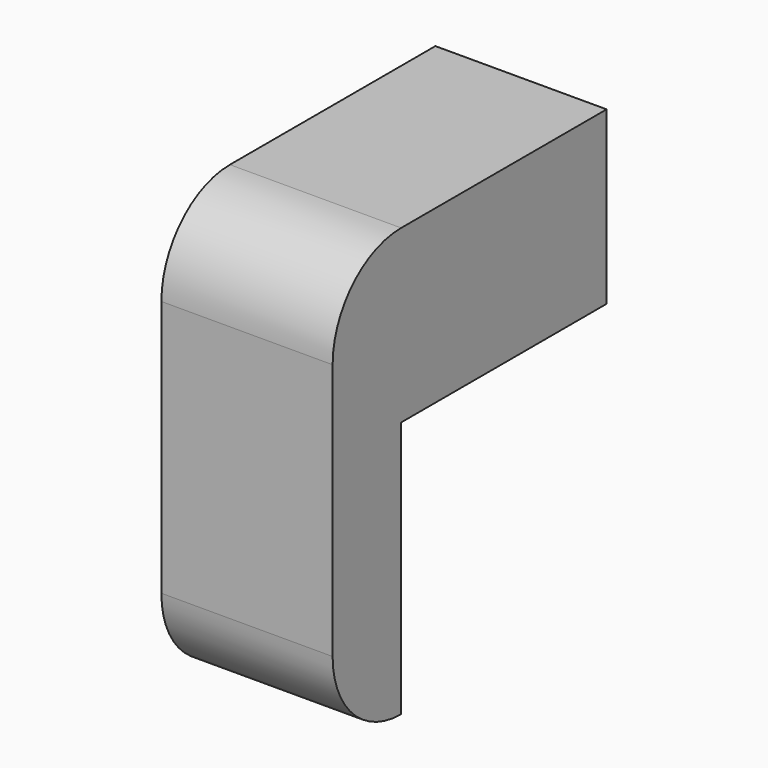
from build123d import *

# Parameters (mm, degrees)
F0_W     = 5.08
F0_H     = 5.08
F1_DEPTH = 7.62
F2_W     = 5.08
F2_H     = 12.7
F3_DEPTH = 2.54
F4_R     = 2.53999


# Not quite as in the source:
# - a fillet or chamfer is up to 0.001 mm smaller than in the source, because OpenCascade refuses the exact size


with BuildPart() as f1:
    # F0 (on Front) → F1 (new body)
    with BuildSketch(Plane.XZ):
        Rectangle(F0_W, F0_H)
    extrude(amount=F1_DEPTH)

    # F2 (on face) → F3 (join)
    with BuildSketch(Plane.XZ.offset(7.62)):
        with Locations((0, -3.81)):
            Rectangle(F2_W, F2_H)
    extrude(amount=F3_DEPTH)

    # F4 (radius 2.54 in the source; OpenCascade refuses exactly that, so slightly less here)
    f4_edges = [f1.edges().sort_by_distance(p)[0] for p in [
        (0, -10.16, 2.54),
        (0, -10.16, -10.16),
    ]]
    fillet(f4_edges, radius=F4_R)


solid = f1.part
